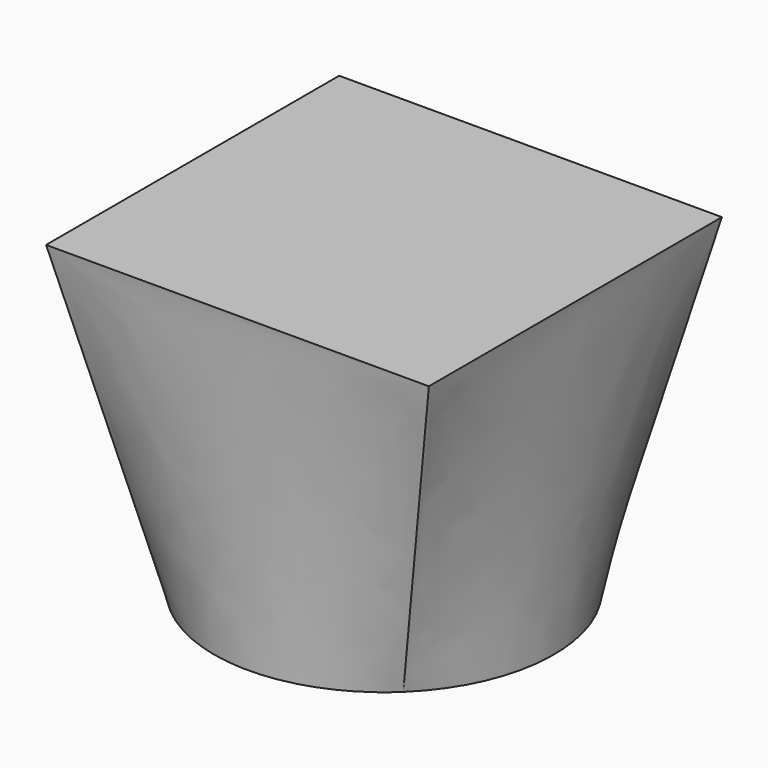
from build123d import *

# Parameters (mm, degrees)
F2_W = 61.2098313868
F2_H = 58.5865564644


# Not quite as in the source:
# - the arcs of a loft's sections are written as splines that run evenly, so that the points pair up as in the source's solid


with BuildPart() as f3:
    # F0 (on Top) → F3 section 0
    with BuildSketch(Plane.XY):
        with BuildLine():
            add(Edge.make_bspline(
                [(19.6305017595, 18.7891956848), (18.4007517777, 20.0740090205), (17.0444922643, 21.2376737801), (14.1309416079, 23.2781011556), (12.5737225081, 24.154813318), (9.3180872769, 25.5876289179), (7.6197516474, 26.1436969262), (4.1471440775, 26.9138384505), (2.3729580041, 27.1278929231), (-1.1831715431, 27.2057642649), (-2.9650270846, 27.0695792085), (-6.4680185448, 26.4521878158), (-8.1890678452, 25.9709967457), (-11.5043032211, 24.6820686235), (-13.098407321, 23.8743634427), (-16.0984839763, 21.9634313758), (-17.5043823491, 20.8602517414), (-18.7891956848, 19.6305017595)],
                knots=[0, 0, 0, 0, 0.125, 0.125, 0.25, 0.25, 0.375, 0.375, 0.5, 0.5, 0.625, 0.625, 0.75, 0.75, 0.875, 0.875, 1, 1, 1, 1], degree=3))
            add(Edge.make_bspline(
                [(-18.7891956848, 19.6305017595), (-20.0740090205, 18.4007517777), (-21.2376737801, 17.0444922643), (-23.2781011556, 14.1309416079), (-24.154813318, 12.5737225081), (-25.5876289179, 9.3180872769), (-26.1436969262, 7.6197516474), (-26.9138384505, 4.1471440775), (-27.1278929231, 2.3729580041), (-27.2057642649, -1.1831715431), (-27.0695792085, -2.9650270846), (-26.4521878158, -6.4680185448), (-25.9709967457, -8.1890678452), (-24.6820686235, -11.5043032211), (-23.8743634427, -13.098407321), (-21.9634313758, -16.0984839763), (-20.8602517414, -17.5043823491), (-19.6305017595, -18.7891956848)],
                knots=[0, 0, 0, 0, 0.125, 0.125, 0.25, 0.25, 0.375, 0.375, 0.5, 0.5, 0.625, 0.625, 0.75, 0.75, 0.875, 0.875, 1, 1, 1, 1], degree=3))
            add(Edge.make_bspline(
                [(-19.6305017595, -18.7891956848), (-18.4007517777, -20.0740090205), (-17.0444922643, -21.2376737801), (-14.1309416079, -23.2781011556), (-12.5737225081, -24.154813318), (-9.3180872769, -25.5876289179), (-7.6197516474, -26.1436969262), (-4.1471440775, -26.9138384505), (-2.3729580041, -27.1278929231), (1.1831715431, -27.2057642649), (2.9650270846, -27.0695792085), (6.4680185448, -26.4521878158), (8.1890678452, -25.9709967457), (11.5043032211, -24.6820686235), (13.098407321, -23.8743634427), (16.0984839763, -21.9634313758), (17.5043823491, -20.8602517414), (18.7891956848, -19.6305017595)],
                knots=[0, 0, 0, 0, 0.125, 0.125, 0.25, 0.25, 0.375, 0.375, 0.5, 0.5, 0.625, 0.625, 0.75, 0.75, 0.875, 0.875, 1, 1, 1, 1], degree=3))
            add(Edge.make_bspline(
                [(18.7891956848, -19.6305017595), (20.0740090205, -18.4007517777), (21.2376737801, -17.0444922643), (23.2781011556, -14.1309416079), (24.154813318, -12.5737225081), (25.5876289179, -9.3180872769), (26.1436969262, -7.6197516474), (26.9138384505, -4.1471440775), (27.1278929231, -2.3729580041), (27.2057642649, 1.1831715431), (27.0695792085, 2.9650270846), (26.4521878158, 6.4680185448), (25.9709967457, 8.1890678452), (24.6820686235, 11.5043032211), (23.8743634427, 13.098407321), (21.9634313758, 16.0984839763), (20.8602517414, 17.5043823491), (19.6305017595, 18.7891956848)],
                knots=[0, 0, 0, 0, 0.125, 0.125, 0.25, 0.25, 0.375, 0.375, 0.5, 0.5, 0.625, 0.625, 0.75, 0.75, 0.875, 0.875, 1, 1, 1, 1], degree=3))
        make_face()
    # F2 (on offset) → F3 section 1
    with BuildSketch(Plane.XY.offset(50.8)):
        Rectangle(F2_W, F2_H)
    loft(ruled=True)


solid = f3.part
